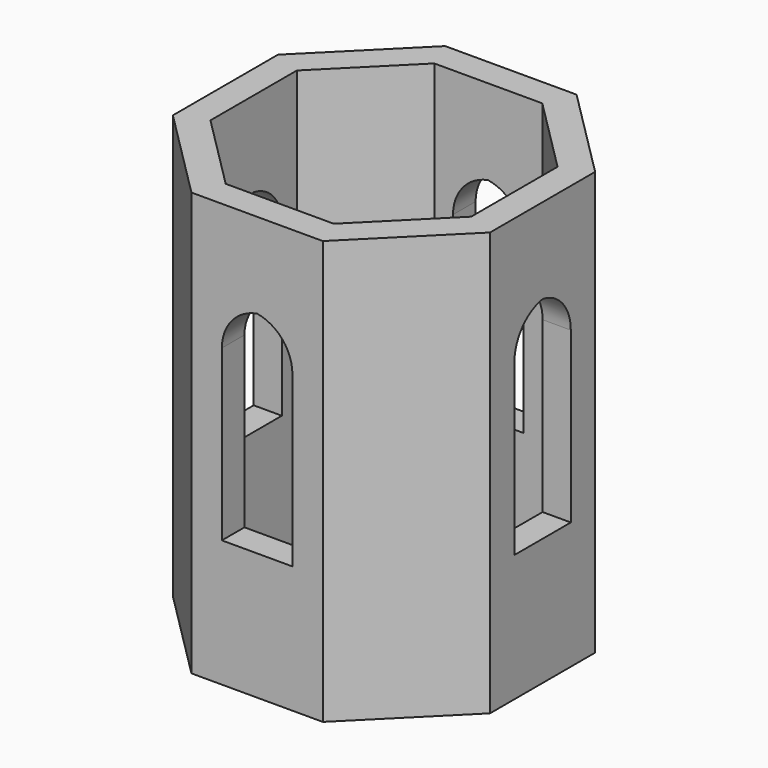
from build123d import *

# Parameters (mm, degrees)
F2_DEPTH      = 3000
F4_START      = -600
F3_W          = 600
F3_H          = 500
F4_DEPTH      = 1500
F3_W_2        = 500
F3_H_2        = 600
F5_T1_DEPTH   = 2100
F5_2_T1_DEPTH = 2100
F5_3_T1_DEPTH = 2100
F5_4_T1_DEPTH = 2100


# Not quite as in the source:
# - a fillet or chamfer that OpenCascade refuses, or shapes differently, is made with other operations: its cross-section is extruded or revolved along the edge and cut away or added
# - a feature names something its author has since deleted; it is built from what else it names


with BuildPart() as f2:
    # F1 (on Top) → F2 (new body)
    with BuildSketch(Plane.XY):
        Polygon((1123.8795325113, 465.5261448397), (465.5261448397, 1123.8795325113), (-465.5261448397, 1123.8795325113), (-1123.8795325113, 465.5261448397), (-1123.8795325113, -465.5261448397), (-465.5261448397, -1123.8795325113), (465.5261448397, -1123.8795325113), (1123.8795325113, -465.5261448397), align=None)
        Polygon((-923.8795325113, 382.6834323651), (-382.6834323651, 923.8795325113), (382.6834323651, 923.8795325113), (923.8795325113, 382.6834323651), (923.8795325113, -382.6834323651), (382.6834323651, -923.8795325113), (-382.6834323651, -923.8795325113), (-923.8795325113, -382.6834323651), align=None, mode=Mode.SUBTRACT)
    extrude(amount=F2_DEPTH)


with BuildPart() as f4:
    # F3 (on face) → F4 (new body)
    with BuildSketch(Plane.XY.offset(3000).offset(F4_START)):
        with Locations((1100, 0)):
            Rectangle(F3_W, F3_H)
    extrude(amount=-F4_DEPTH)

    # F5#4: fillet of radius 300 on 2 edges, made by hand

    # F5_4_s2 → F5_4_t1 (cut)
    with BuildSketch(Plane.YZ.offset(50)):
        with BuildLine():
            ThreePointArc((-250, 2100), (-162.132034356, 2312.132034356), (50, 2400))
            Line((50, 2400), (-250, 2400))
            Line((-250, 2400), (-250, 2100))
        make_face()
        with BuildLine():
            ThreePointArc((250, 2100), (162.132034356, 2312.132034356), (-50, 2400))
            Line((-50, 2400), (250, 2400))
            Line((250, 2400), (250, 2100))
        make_face()
    extrude(amount=F5_4_T1_DEPTH, mode=Mode.SUBTRACT)


with BuildPart() as f4b:
    # F3 (on face) → F4, piece 2 (new body)
    with BuildSketch(Plane.XY.offset(3000).offset(F4_START)):
        with Locations((0, 1100)):
            Rectangle(F3_W_2, F3_H_2)
    extrude(amount=-F4_DEPTH)

    # F5: fillet of radius 300 on 2 edges, made by hand

    # F5_s2 → F5_t1 (cut)
    with BuildSketch(Plane.XZ.offset(-2150)):
        with BuildLine():
            ThreePointArc((-250, 2100), (-162.132034356, 2312.132034356), (50, 2400))
            Line((50, 2400), (-250, 2400))
            Line((-250, 2400), (-250, 2100))
        make_face()
        with BuildLine():
            ThreePointArc((250, 2100), (162.132034356, 2312.132034356), (-50, 2400))
            Line((-50, 2400), (250, 2400))
            Line((250, 2400), (250, 2100))
        make_face()
    extrude(amount=F5_T1_DEPTH, mode=Mode.SUBTRACT)


with BuildPart() as f4c:
    # F3 (on face) → F4, piece 3 (new body)
    with BuildSketch(Plane.XY.offset(3000).offset(F4_START)):
        with Locations((-1100, 0)):
            Rectangle(F3_W, F3_H)
    extrude(amount=-F4_DEPTH)

    # F5#2: fillet of radius 300 on 2 edges, made by hand

    # F5_2_s2 → F5_2_t1 (cut)
    with BuildSketch(Plane.YZ.offset(-2150)):
        with BuildLine():
            ThreePointArc((250, 2100), (162.132034356, 2312.132034356), (-50, 2400))
            Line((-50, 2400), (250, 2400))
            Line((250, 2400), (250, 2100))
        make_face()
        with BuildLine():
            ThreePointArc((-250, 2100), (-162.132034356, 2312.132034356), (50, 2400))
            Line((50, 2400), (-250, 2400))
            Line((-250, 2400), (-250, 2100))
        make_face()
    extrude(amount=F5_2_T1_DEPTH, mode=Mode.SUBTRACT)


with BuildPart() as f4d:
    # F3 (on face) → F4, piece 4 (new body)
    with BuildSketch(Plane.XY.offset(3000).offset(F4_START)):
        with Locations((0, -1100)):
            Rectangle(F3_W_2, F3_H_2)
    extrude(amount=-F4_DEPTH)

    # F5#3: fillet of radius 300 on 2 edges, made by hand

    # F5_3_s2 → F5_3_t1 (cut)
    with BuildSketch(Plane.XZ.offset(50)):
        with BuildLine():
            ThreePointArc((-250, 2100), (-162.132034356, 2312.132034356), (50, 2400))
            Line((50, 2400), (-250, 2400))
            Line((-250, 2400), (-250, 2100))
        make_face()
        with BuildLine():
            ThreePointArc((250, 2100), (162.132034356, 2312.132034356), (-50, 2400))
            Line((-50, 2400), (250, 2400))
            Line((250, 2400), (250, 2100))
        make_face()
    extrude(amount=F5_3_T1_DEPTH, mode=Mode.SUBTRACT)


with BuildPart() as f2_1:
    add(f2.part)

    # F6: cut F4, F4b, F4c, F4d
    add(f4.part, mode=Mode.SUBTRACT)
    add(f4b.part, mode=Mode.SUBTRACT)
    add(f4c.part, mode=Mode.SUBTRACT)
    add(f4d.part, mode=Mode.SUBTRACT)


solid = f2_1.part
